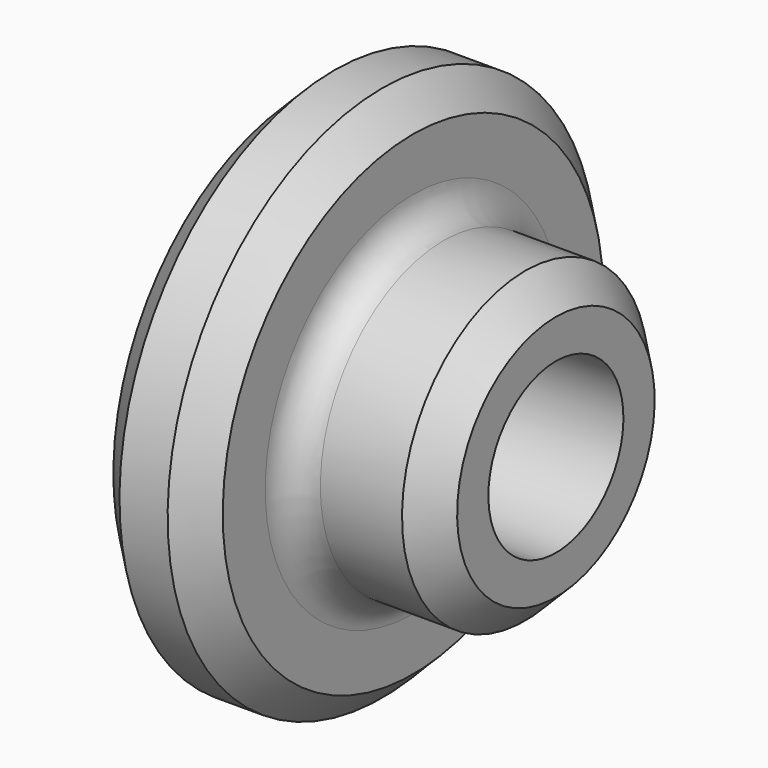
from build123d import *

# Parameters (mm, degrees)
F2_R    = 5.08
F3_SIZE = 5.08


# Not quite as in the source:
# - the program builds the solid bodies; features that only make, move or delete a surface that nothing else refers to are left out


with BuildPart() as f1:
    # F0 (on Front) → F1 (revolve)
    with BuildSketch(Plane.XZ):
        Polygon((18.1504152715, 44.5240847766), (0, 44.5240847766), (0, 14.0017503873), (41.8570823967, 14.0017503873), (41.8570823967, 25.5587510765), (18.1504152715, 25.5587510765), align=None)
    revolve(axis=Axis((21.6693747789, 0, 0), (1, 0, 0)))

    # F2
    f2_edges = [f1.edges().sort_by_distance(p)[0] for p in [
        (18.150415, 0, -25.558751),
    ]]
    fillet(f2_edges, radius=F2_R)

    # F3
    f3_edges = [f1.edges().sort_by_distance(p)[0] for p in [
        (41.857082, 0, -25.558751),
        (18.150415, 0, -44.524085),
        (0, 0, -44.524085),
    ]]
    chamfer(f3_edges, length=F3_SIZE)


solid = f1.part
